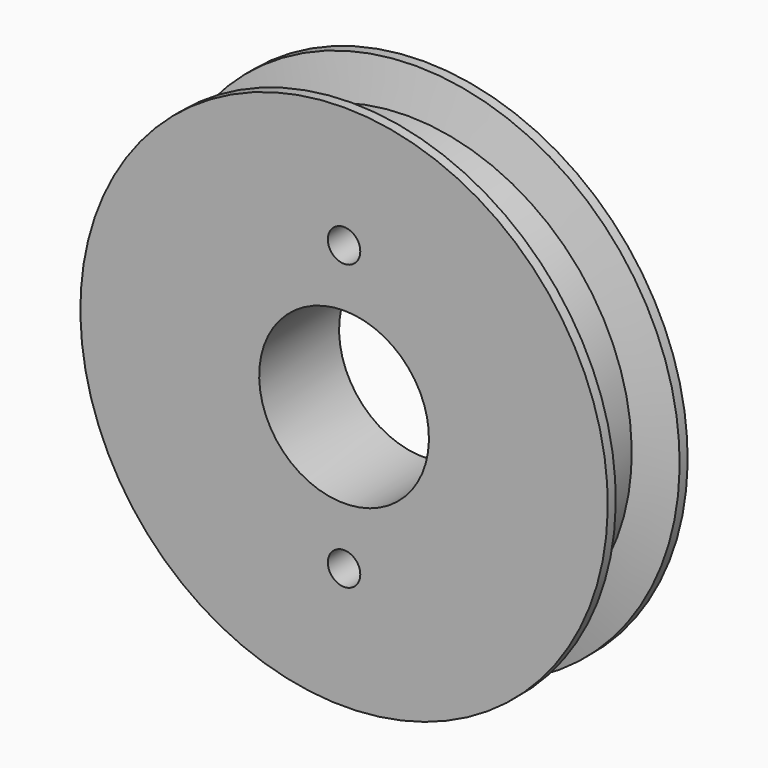
from build123d import *

# Parameters (mm, degrees)
F2_SIZE2       = 1.58749
F2_SIZE        = 6.34999
F3_SIZE2       = 1.58749
F3_SIZE        = 6.34999
F5_D           = 5.159375
F5_CSINK_D     = 11.1125
F5_CSINK_ANGLE = 90


# Not quite as in the source:
# - a fillet or chamfer is up to 0.001 mm smaller than in the source, because OpenCascade refuses the exact size


with BuildPart() as f1:
    # F0 (on Right) → F1 (revolve)
    with BuildSketch(Plane.YZ):
        Polygon((-15.875, 13.49375), (0, 13.49375), (0, 41.9197008275), (-3.175, 41.9197008275), (-3.175, 35.5697008275), (-12.7, 35.5697008275), (-12.7, 41.9197008275), (-15.875, 41.9197008275), align=None)
    revolve(axis=Axis((0, -7.9375, 0), (0, 1, 0)))

    # F2 (size 6.35 and 1.5875 in the source; OpenCascade refuses exactly that, so slightly less here)
    f2_edges = [f1.edges().sort_by_distance(p)[0] for p in [
        (0, -12.7, -41.919701),
    ]]
    f2_side = f1.faces().sort_by_distance((0, -12.7, -36.755369))[0]
    chamfer(f2_edges, length=F2_SIZE, length2=F2_SIZE2, reference=f2_side)

    # F3 (size 6.35 and 1.5875 in the source; OpenCascade refuses exactly that, so slightly less here)
    f3_edges = [f1.edges().sort_by_distance(p)[0] for p in [
        (0, -3.175, -41.919701),
    ]]
    chamfer(f3_edges, length=F3_SIZE, length2=F3_SIZE2)

    # F5 (through all)
    with Locations(Plane(origin=(0, 0, 0), x_dir=(-1, 0, 0), z_dir=(0, 1, 0))):
        with Locations((0, 22.606), (0, -22.606)):
            CounterSinkHole(F5_D / 2, F5_CSINK_D / 2, counter_sink_angle=F5_CSINK_ANGLE)


solid = f1.part
